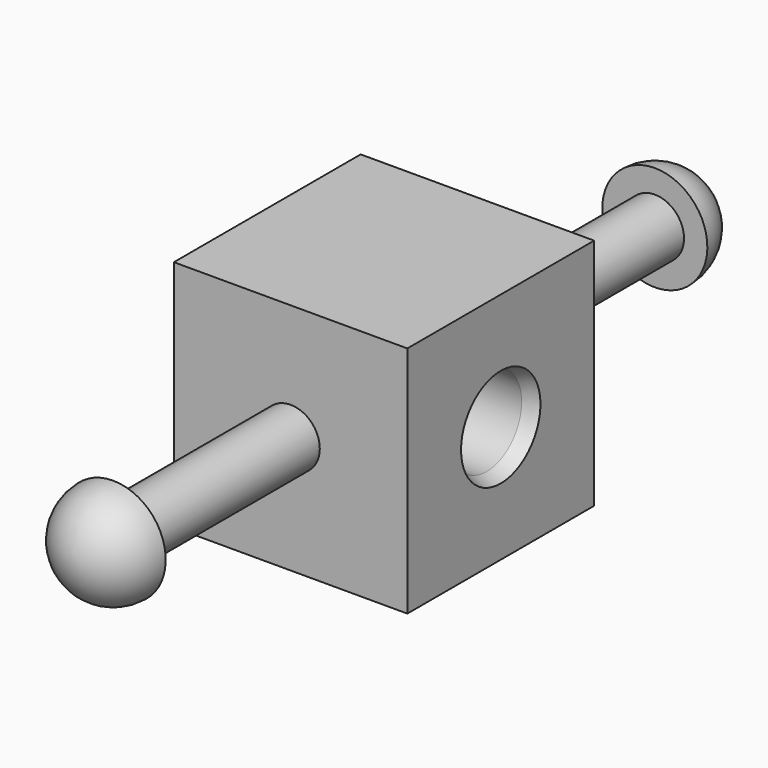
from build123d import *

# Parameters (mm, degrees)
F0_W           = 25.4
F0_H           = 25.4
F1_DEPTH       = 12.7
F3_D           = 9.525
F3_CSINK_D     = 10.795
F3_CSINK_ANGLE = 45
F5_R           = 3.175
F6_DEPTH       = 24.13


# Not quite as in the source:
# - a pattern or mirror of a feature is missing from the dataset's text; its kind, count and spacing are read off the source's solid


with BuildPart() as f1:
    # F0 (on Right) → F1 (new body)
    with BuildSketch(Plane.YZ):
        Rectangle(F0_W, F0_H)
    extrude(amount=-F1_DEPTH)

    # F3 (through all)
    with Locations(Plane.YZ):
        with Locations((0, 0)):
            CounterSinkHole(F3_D / 2, F3_CSINK_D / 2, counter_sink_angle=F3_CSINK_ANGLE)

    # F4: F1 across face


with BuildPart() as f1_1:
    add(f1.part)
    add(f1.part.mirror(Plane(origin=(-12.7, 0, 0), x_dir=(0, 1, 0), z_dir=(-1, 0, 0))))

    # F5 (on face) → F6 (join)
    with BuildSketch(Plane.XZ.offset(12.7)):
        with Locations((-12.7, 0)):
            Circle(F5_R)
    f6 = extrude(amount=F6_DEPTH)

    # F6_copies: F6 across plane
    add(f6.mirror(Plane.ZX))

    # F8 (on offset) → F9 (revolve)
    with BuildSketch(Plane(origin=(-12.7, 0, 0), x_dir=(0, -1, 0), z_dir=(-1, 0, 0))):
        with BuildLine():
            Line((36.83, 5.715), (36.83, 3.175))
            Line((36.83, 3.175), (36.83, 0))
            Line((36.83, 0), (42.545, 0))
            ThreePointArc((42.545, 0), (40.8711152545, 4.0411152545), (36.83, 5.715))
        make_face()
    f9 = revolve(axis=Axis((-12.7, -39.6875, 0), (0, 1, 0)))

    # F9_copies: F9 across plane
    add(f9.mirror(Plane.ZX))


solid = f1_1.part
